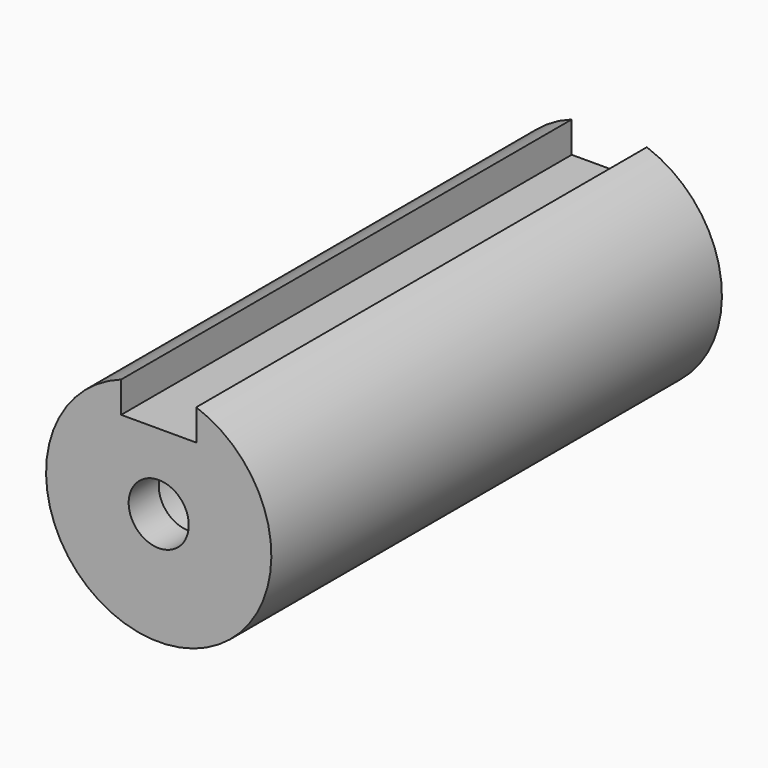
from build123d import *

# Parameters (mm, degrees)
F0_R      = 6
F1_DEPTH  = 30
F2_R      = 2.75
F3_DEPTH  = 30.001
F8_R      = 5
F8_R_2    = 1.6
F9_DEPTH  = 2
F12_W     = 4
F12_H     = 30
F13_DEPTH = 3


with BuildPart() as f1:
    # F0 (on Front) → F1 (new body)
    with BuildSketch(Plane.XZ):
        Circle(F0_R)
    extrude(amount=F1_DEPTH)

    # F2 (on face) → F3 (cut, through all)
    with BuildSketch(Plane.XZ.offset(30)):
        Circle(F2_R)
    extrude(amount=-F3_DEPTH, mode=Mode.SUBTRACT)

    # F8 (on face) → F9 (join)
    with BuildSketch(Plane.XZ.offset(30)):
        Circle(F8_R)
        Circle(F8_R_2, mode=Mode.SUBTRACT)
    extrude(amount=-F9_DEPTH)

    # F12 (on offset) → F13 (cut)
    with BuildSketch(Plane.XY.offset(4)):
        with Locations((0, -15)):
            Rectangle(F12_W, F12_H)
    extrude(amount=F13_DEPTH, mode=Mode.SUBTRACT)


solid = f1.part
